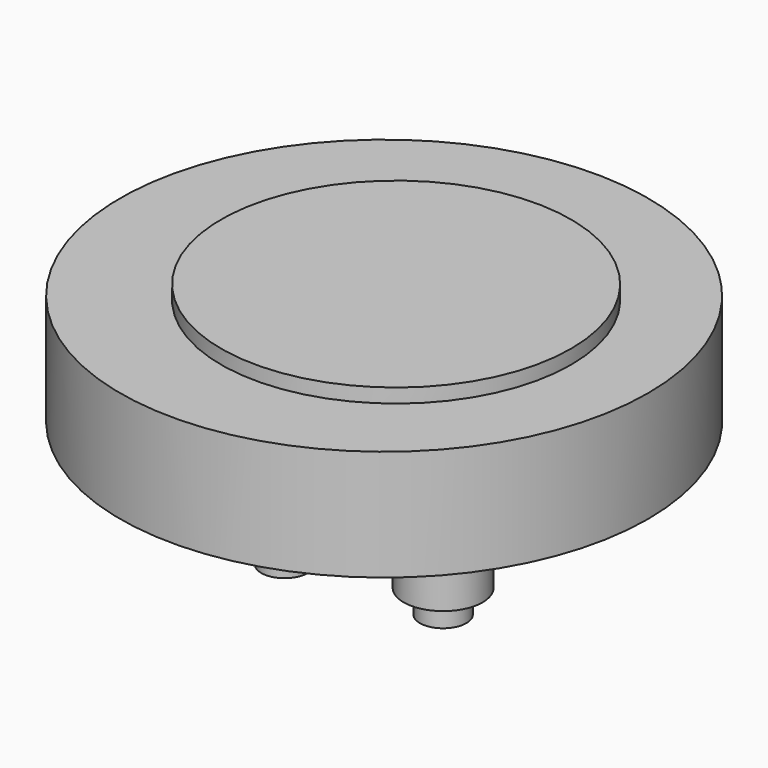
from build123d import *

# Parameters (mm, degrees)
F0_R      = 284.48
F0_R_2    = 107.1929715192
F0_R_3    = 113.5568544934
F1_DEPTH  = 43.18
F2_DEPTH  = 25.4
F3_R      = 188.583728209
F4_DEPTH  = 83.82
F5_R      = 191.3062955449
F6_DEPTH  = 25.4
F7_DEPTH  = 50.8
F8_R      = 44.4860383671
F8_R_2    = 42.5130720405
F9_DEPTH  = 73.66
F11_R     = 25.0558665745
F12_DEPTH = 96.52
F13_R     = 24.5435955791
F15_DEPTH = 60.96
F16_R     = 25.0526065755
F17_DEPTH = 25.4
F18_R     = 25.0571
F18_R_2   = 24.5435955791
F19_DEPTH = 25.4


# Not quite as in the source:
# - the program builds the solid bodies; features that only make, move or delete a surface that nothing else refers to are left out


with BuildPart() as f1:
    # F0 (on Top) → F1 (new body)
    with BuildSketch(Plane.XY):
        Circle(F0_R)
        with Locations((-137.995660305, 0)):
            Circle(F0_R_2, mode=Mode.SUBTRACT)
        with Locations((127.078294754, 0)):
            Circle(F0_R_3, mode=Mode.SUBTRACT)
        with BuildLine():
            ThreePointArc((-102.7708947659, 136.166498065), (-10.3978756011, 204.9943768322), (94.8023349047, 158.0585986376))
            ThreePointArc((94.8023349047, 158.0585986376), (-4.0832297138, 148.0055566847), (-102.7708947659, 136.166498065))
        make_face(mode=Mode.SUBTRACT)
        with Locations((-137.995660305, 0)):
            Circle(F0_R_2)
        with Locations((127.078294754, 0)):
            Circle(F0_R_3)
        with BuildLine():
            ThreePointArc((-102.7708947659, 136.166498065), (-4.0832297138, 148.0055566847), (94.8023349047, 158.0585986376))
            ThreePointArc((94.8023349047, 158.0585986376), (-10.3978756011, 204.9943768322), (-102.7708947659, 136.166498065))
        make_face()
    extrude(amount=F1_DEPTH)

    # F2 (add): a face of the model
    f2_faces = [f1.faces().sort_by_distance(p)[0] for p in [
        (0, 0, 0),
    ]]
    extrude(f2_faces, amount=F2_DEPTH)

    # F3 (on face) → F4 (join)
    with BuildSketch(Plane(origin=(0, 0, -25.4), x_dir=(1, 0, 0), z_dir=(0, 0, -1))):
        with Locations((12.9366638139, 0)):
            Circle(F3_R)
    extrude(amount=-F4_DEPTH)

    # F5 (on face) → F6 (join)
    with BuildSketch(Plane(origin=(0, 0, -25.4), x_dir=(1, 0, 0), z_dir=(0, 0, -1))):
        with Locations((18.2807631791, 0)):
            Circle(F5_R)
    extrude(amount=F6_DEPTH)

    # F7 (add): faces of the model
    f7_faces = [f1.faces().sort_by_distance(p)[0] for p in [
        (-276.4336905155, 0, -25.4),
        (-173.3657778507, 0, -25.4),
        (18.2807631791, 0, -50.8),
    ]]
    extrude(f7_faces, amount=F7_DEPTH)

    # F8 (on face) → F9 (join)
    with BuildSketch(Plane(origin=(0, 0, -101.6), x_dir=(1, 0, 0), z_dir=(0, 0, -1))):
        with Locations((-52.0154200494, 69.075293839)):
            Circle(F8_R)
        with Locations((109.2234924436, 57.04626441)):
            Circle(F8_R_2)
    extrude(amount=F9_DEPTH)

    # F11 (on face) → F12 (join)
    with BuildSketch(Plane(origin=(0, 0, -175.26), x_dir=(1, 0, 0), z_dir=(0, 0, -1))):
        with Locations((-52.0154200494, 69.075293839)):
            Circle(F11_R)
    extrude(amount=-F12_DEPTH)

    # F13 (on face) → F15 (join)
    with BuildSketch(Plane(origin=(0, 0, -175.26), x_dir=(1, 0, 0), z_dir=(0, 0, -1))):
        with Locations((-52.0154200494, 69.075293839)):
            Circle(F13_R)
    extrude(amount=-F15_DEPTH)

    # F16 (on face) → F17 (join)
    with BuildSketch(Plane(origin=(0, 0, -175.26), x_dir=(1, 0, 0), z_dir=(0, 0, -1))):
        with Locations((109.2234924436, 57.04626441)):
            Circle(F16_R)
    extrude(amount=F17_DEPTH)

    # F18 (on face) → F19 (join)
    with BuildSketch(Plane(origin=(0, 0, -175.26), x_dir=(1, 0, 0), z_dir=(0, 0, -1))):
        with Locations((-52.0154200494, 69.075293839)):
            Circle(F18_R)
        with Locations((-52.0154200494, 69.075293839)):
            Circle(F18_R_2, mode=Mode.SUBTRACT)
        with Locations((-52.0154200494, 69.075293839)):
            Circle(F18_R_2)
    extrude(amount=F19_DEPTH)


solid = f1.part
